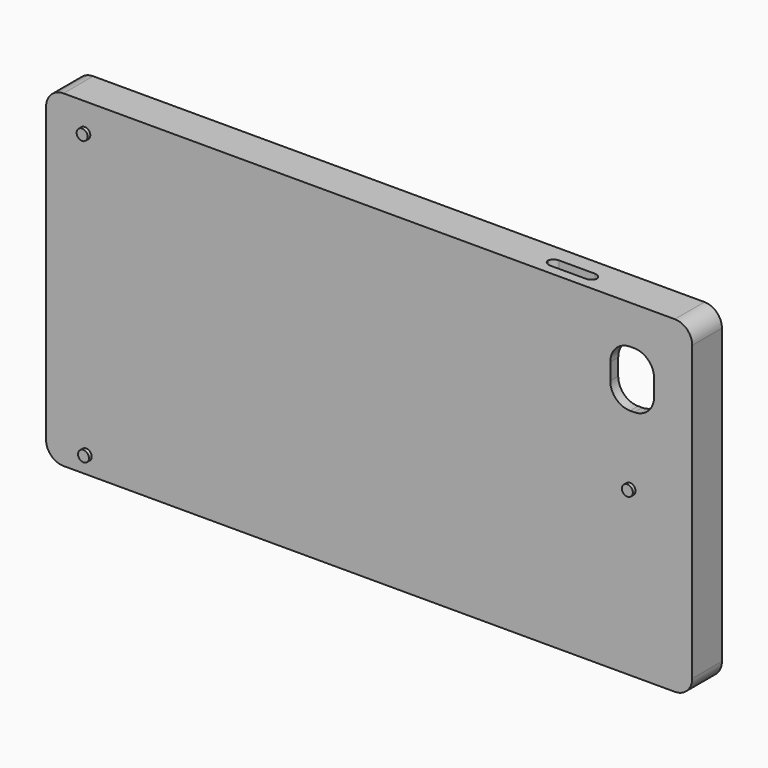
from build123d import *

# Parameters (mm, degrees)
F0_W         = 160.02
F0_H         = 78.74
F1_DEPTH     = 6.94228
F2_T         = 2.54
F3_T1_DEPTH  = 6.94228
F3_T3_DEPTH  = 31.70728
F4_W         = 11.2012028694
F4_H         = 14.4015364349
F6_DEPTH     = 25.4
F7_R         = 5.08
F8_W         = 2.54
F8_H         = 12.7
F8_H_2       = 17.78
F9_DEPTH     = 25.4
F10_W        = 10.3627294302
F10_H        = 4.2195547159
F10_W_2      = 10.414
F10_H_2      = 3.1508285339
F11_DEPTH    = 25.4
F12_T1_DEPTH = 2.54
F12_T3_DEPTH = 2.54
F13_W        = 12.7
F13_H        = 2.8448
F14_DEPTH    = 25.4
F15_T1_DEPTH = 2.54
F16_R        = 1.397
F17_DEPTH    = 0.86535


# Not quite as in the source:
# - a fillet or chamfer that OpenCascade refuses, or shapes differently, is made with other operations: its cross-section is extruded or revolved along the edge and cut away or added


with BuildPart() as f1:
    # F0 (on Front) → F1 (new body)
    with BuildSketch(Plane.XZ):
        with Locations((-0.5110458827, -0.4783872414)):
            Rectangle(F0_W, F0_H)
    extrude(amount=F1_DEPTH)

    # F2
    f2_openings = [f1.faces().sort_by_distance(p)[0] for p in [
        (-0.511046, 0, -0.478387),
    ]]
    offset(amount=F2_T, openings=f2_openings, kind=Kind.INTERSECTION)

    # F3: fillet of radius 4.445 on 8 edges, made by hand

    # F3_s2 → F3_t1 (join)
    with BuildSketch(Plane.XZ):
        with BuildLine():
            ThreePointArc((-76.0760458827, 38.8916127586), (-79.2191355251, 37.589702401), (-80.5210458827, 34.4466127586))
            Line((-80.5210458827, 34.4466127586), (-80.5210458827, 38.8916127586))
            Line((-80.5210458827, 38.8916127586), (-76.0760458827, 38.8916127586))
        make_face()
        with BuildLine():
            ThreePointArc((-80.5210458827, -35.4033872414), (-79.2191355251, -38.5464768837), (-76.0760458827, -39.8483872414))
            Line((-76.0760458827, -39.8483872414), (-80.5210458827, -39.8483872414))
            Line((-80.5210458827, -39.8483872414), (-80.5210458827, -35.4033872414))
        make_face()
        with BuildLine():
            ThreePointArc((79.4989541173, -35.4033872414), (78.1970437597, -38.5464768837), (75.0539541173, -39.8483872414))
            Line((75.0539541173, -39.8483872414), (79.4989541173, -39.8483872414))
            Line((79.4989541173, -39.8483872414), (79.4989541173, -35.4033872414))
        make_face()
        with BuildLine():
            ThreePointArc((79.4989541173, 34.4466127586), (78.1970437597, 37.589702401), (75.0539541173, 38.8916127586))
            Line((75.0539541173, 38.8916127586), (79.4989541173, 38.8916127586))
            Line((79.4989541173, 38.8916127586), (79.4989541173, 34.4466127586))
        make_face()
    extrude(amount=F3_T1_DEPTH)

    # F3_s4 → F3_t3 (cut)
    with BuildSketch(Plane.XZ.offset(-11.1125)):
        with BuildLine():
            ThreePointArc((77.5939541173, -42.3883872414), (80.7370437597, -41.0864768837), (82.0389541173, -37.9433872414))
            Line((82.0389541173, -37.9433872414), (82.0389541173, -42.3883872414))
            Line((82.0389541173, -42.3883872414), (77.5939541173, -42.3883872414))
        make_face()
        with BuildLine():
            ThreePointArc((82.0389541173, 36.9866127586), (80.7370437597, 40.129702401), (77.5939541173, 41.4316127586))
            Line((77.5939541173, 41.4316127586), (82.0389541173, 41.4316127586))
            Line((82.0389541173, 41.4316127586), (82.0389541173, 36.9866127586))
        make_face()
        with BuildLine():
            ThreePointArc((-83.0610458827, 36.9866127586), (-81.7591355251, 40.129702401), (-78.6160458827, 41.4316127586))
            Line((-78.6160458827, 41.4316127586), (-83.0610458827, 41.4316127586))
            Line((-83.0610458827, 41.4316127586), (-83.0610458827, 36.9866127586))
        make_face()
        with BuildLine():
            ThreePointArc((-83.0610458827, -37.9433872414), (-81.7591355251, -41.0864768837), (-78.6160458827, -42.3883872414))
            Line((-78.6160458827, -42.3883872414), (-83.0610458827, -42.3883872414))
            Line((-83.0610458827, -42.3883872414), (-83.0610458827, -37.9433872414))
        make_face()
    extrude(amount=F3_T3_DEPTH, mode=Mode.SUBTRACT)

    # F4 (on face) → F6 (cut)
    with BuildSketch(Plane(origin=(0, -6.94228, 0), x_dir=(-1, 0, 0), z_dir=(0, 1, 0))):
        with Locations((-66.6961297393, 24.3242625147)):
            Rectangle(F4_W, F4_H)
    extrude(amount=-F6_DEPTH, mode=Mode.SUBTRACT)

    # F7
    f7_edges = [f1.edges().sort_by_distance(p)[0] for p in [
        (72.296731, -8.21228, 31.525031),
        (72.296731, -8.21228, 17.123494),
        (61.095528, -8.21228, 31.525031),
        (61.095528, -8.21228, 17.123494),
    ]]
    fillet(f7_edges, radius=F7_R)

    # F8 (on face) → F9 (cut)
    with BuildSketch(Plane(origin=(-83.0610458827, 0, 0), x_dir=(0, -1, 0), z_dir=(-1, 0, 0))):
        with BuildLine():
            ThreePointArc((3.9402758845, -24.4620272314), (3.5303106613, -28.2545002504), (6.90014, -26.4669954777))
            ThreePointArc((6.90014, -26.4669954777), (6.5286447728, -25.256166139), (5.5420041155, -24.4620272314))
            ThreePointArc((5.5420041155, -24.4620272314), (4.74114, -24.7671066221), (3.9402758845, -24.4620272314))
        make_face()
        with BuildLine():
            ThreePointArc((3.9402758845, -24.4620272314), (4.74114, -24.3079954777), (5.5420041155, -24.4620272314))
            ThreePointArc((5.5420041155, -24.4620272314), (5.8395341143, -24.0557928593), (5.9448541617, -23.5633924603))
            ThreePointArc((5.9448541617, -23.5633924603), (4.2487396011, -22.4649983461), (3.9402758845, -24.4620272314))
        make_face()
        with Locations((4.74114, 0)):
            Rectangle(F8_W, F8_H)
        with Locations((4.74114, 20.6036127586)):
            Rectangle(F8_W, F8_H_2)
    extrude(amount=-F9_DEPTH, mode=Mode.SUBTRACT)

    # F10 (on face) → F11 (cut)
    with BuildSketch(Plane(origin=(0, 0, -42.3883872414), x_dir=(1, 0, 0), z_dir=(0, 0, -1))):
        with Locations((46.1594350636, 4.74114)):
            Rectangle(F10_W, F10_H)
        with Locations((27.6780048452, 4.74114)):
            Rectangle(F10_W_2, F10_H_2)
        with Locations((13.9850524713, 4.74114)):
            Rectangle(F10_W_2, F10_H_2)
    extrude(amount=-F11_DEPTH, mode=Mode.SUBTRACT)

    # F12: fillet of radius 1.5288490226 on 20 edges, made by hand

    # F12_s2 → F12_t1 (join)
    with BuildSketch(Plane.XY.offset(-42.3883872414)):
        with BuildLine():
            ThreePointArc((19.1920524713, -4.7877052443), (18.7442629599, -5.8687647556), (17.6632034486, -6.316554267))
            Line((17.6632034486, -6.316554267), (19.1920524713, -6.316554267))
            Line((19.1920524713, -6.316554267), (19.1920524713, -4.7877052443))
        make_face()
        with BuildLine():
            ThreePointArc((8.7780524713, -4.7877052443), (9.2258419826, -5.8687647556), (10.3069014939, -6.316554267))
            Line((10.3069014939, -6.316554267), (8.7780524713, -6.316554267))
            Line((8.7780524713, -6.316554267), (8.7780524713, -4.7877052443))
        make_face()
        with BuildLine():
            ThreePointArc((10.3069014939, -3.165725733), (9.2258419826, -3.6135152444), (8.7780524713, -4.6945747557))
            Line((8.7780524713, -4.6945747557), (8.7780524713, -3.165725733))
            Line((8.7780524713, -3.165725733), (10.3069014939, -3.165725733))
        make_face()
        with BuildLine():
            ThreePointArc((19.1920524713, -4.6945747557), (18.7442629599, -3.6135152444), (17.6632034486, -3.165725733))
            Line((17.6632034486, -3.165725733), (19.1920524713, -3.165725733))
            Line((19.1920524713, -3.165725733), (19.1920524713, -4.6945747557))
        make_face()
        with BuildLine():
            ThreePointArc((31.3561558226, -6.316554267), (32.4372153339, -5.8687647556), (32.8850048452, -4.7877052443))
            Line((32.8850048452, -4.7877052443), (32.8850048452, -6.316554267))
            Line((32.8850048452, -6.316554267), (31.3561558226, -6.316554267))
        make_face()
        with BuildLine():
            ThreePointArc((32.8850048452, -4.6945747557), (32.4372153339, -3.6135152444), (31.3561558226, -3.165725733))
            Line((31.3561558226, -3.165725733), (32.8850048452, -3.165725733))
            Line((32.8850048452, -3.165725733), (32.8850048452, -4.6945747557))
        make_face()
        with BuildLine():
            ThreePointArc((23.9998538678, -6.316554267), (22.9187943565, -5.8687647556), (22.4710048452, -4.7877052443))
            Line((22.4710048452, -4.7877052443), (22.4710048452, -6.316554267))
            Line((22.4710048452, -6.316554267), (23.9998538678, -6.316554267))
        make_face()
        with BuildLine():
            ThreePointArc((23.9998538678, -3.165725733), (22.9187943565, -3.6135152444), (22.4710048452, -4.6945747557))
            Line((22.4710048452, -4.6945747557), (22.4710048452, -3.165725733))
            Line((22.4710048452, -3.165725733), (23.9998538678, -3.165725733))
        make_face()
        with BuildLine():
            ThreePointArc((51.3407997787, -4.1602116647), (50.8930102674, -3.0791521534), (49.8119507561, -2.631362642))
            Line((49.8119507561, -2.631362642), (51.3407997787, -2.631362642))
            Line((51.3407997787, -2.631362642), (51.3407997787, -4.1602116647))
        make_face()
        with BuildLine():
            ThreePointArc((49.8119507561, -6.850917358), (50.8930102674, -6.4031278466), (51.3407997787, -5.3220683353))
            Line((51.3407997787, -5.3220683353), (51.3407997787, -6.850917358))
            Line((51.3407997787, -6.850917358), (49.8119507561, -6.850917358))
        make_face()
        with BuildLine():
            ThreePointArc((42.5069193711, -6.850917358), (41.4258598598, -6.4031278466), (40.9780703485, -5.3220683353))
            Line((40.9780703485, -5.3220683353), (40.9780703485, -6.850917358))
            Line((40.9780703485, -6.850917358), (42.5069193711, -6.850917358))
        make_face()
        with BuildLine():
            ThreePointArc((42.5069193711, -2.631362642), (41.4258598598, -3.0791521534), (40.9780703485, -4.1602116647))
            Line((40.9780703485, -4.1602116647), (40.9780703485, -2.631362642))
            Line((40.9780703485, -2.631362642), (42.5069193711, -2.631362642))
        make_face()
    extrude(amount=F12_T1_DEPTH)

    # F12_s4 → F12_t3 (join)
    with BuildSketch(Plane.YZ.offset(-83.0610458827)):
        with BuildLine():
            ThreePointArc((-4.9999890226, 11.7136127586), (-3.9189295113, 12.16140227), (-3.47114, 13.2424617813))
            Line((-3.47114, 13.2424617813), (-3.47114, 11.7136127586))
            Line((-3.47114, 11.7136127586), (-4.9999890226, 11.7136127586))
        make_face()
        with BuildLine():
            ThreePointArc((-6.01114, 27.964763736), (-5.5633504887, 29.0458232473), (-4.4822909774, 29.4936127586))
            Line((-4.4822909774, 29.4936127586), (-6.01114, 29.4936127586))
            Line((-6.01114, 29.4936127586), (-6.01114, 27.964763736))
        make_face()
        with BuildLine():
            ThreePointArc((-3.47114, 27.964763736), (-3.9189295113, 29.0458232473), (-4.9999890226, 29.4936127586))
            Line((-4.9999890226, 29.4936127586), (-3.47114, 29.4936127586))
            Line((-3.47114, 29.4936127586), (-3.47114, 27.964763736))
        make_face()
        with BuildLine():
            ThreePointArc((-6.01114, 13.2424617813), (-5.5633504887, 12.16140227), (-4.4822909774, 11.7136127586))
            Line((-4.4822909774, 11.7136127586), (-6.01114, 11.7136127586))
            Line((-6.01114, 11.7136127586), (-6.01114, 13.2424617813))
        make_face()
        with BuildLine():
            ThreePointArc((-6.01114, 4.8211509774), (-5.5633504887, 5.9022104887), (-4.4822909774, 6.35))
            Line((-4.4822909774, 6.35), (-6.01114, 6.35))
            Line((-6.01114, 6.35), (-6.01114, 4.8211509774))
        make_face()
        with BuildLine():
            ThreePointArc((-6.01114, -4.8211509774), (-5.5633504887, -5.9022104887), (-4.4822909774, -6.35))
            Line((-4.4822909774, -6.35), (-6.01114, -6.35))
            Line((-6.01114, -6.35), (-6.01114, -4.8211509774))
        make_face()
        with BuildLine():
            ThreePointArc((-4.9999890226, -6.35), (-3.9189295113, -5.9022104887), (-3.47114, -4.8211509774))
            Line((-3.47114, -4.8211509774), (-3.47114, -6.35))
            Line((-3.47114, -6.35), (-4.9999890226, -6.35))
        make_face()
        with BuildLine():
            ThreePointArc((-3.47114, 4.8211509774), (-3.9189295113, 5.9022104887), (-4.9999890226, 6.35))
            Line((-4.9999890226, 6.35), (-3.47114, 6.35))
            Line((-3.47114, 6.35), (-3.47114, 4.8211509774))
        make_face()
    extrude(amount=F12_T3_DEPTH)

    # F13 (on face) → F14 (cut)
    with BuildSketch(Plane.XY.offset(41.4316127586)):
        with Locations((48.2621807605, -5.5104298601)):
            Rectangle(F13_W, F13_H)
    extrude(amount=-F14_DEPTH, mode=Mode.SUBTRACT)

    # F15: fillet of radius 1.7551815441 on 4 edges, made by hand

    # F15_s2 → F15_t1 (join)
    with BuildSketch(Plane.XY.offset(38.8916127586)):
        with BuildLine():
            ThreePointArc((52.8569992164, -4.0880298601), (54.0980999884, -4.6021106321), (54.6121807605, -5.8432114042))
            Line((54.6121807605, -5.8432114042), (54.6121807605, -4.0880298601))
            Line((54.6121807605, -4.0880298601), (52.8569992164, -4.0880298601))
        make_face()
        with BuildLine():
            ThreePointArc((43.6673623046, -4.0880298601), (42.4262615326, -4.6021106321), (41.9121807605, -5.8432114042))
            Line((41.9121807605, -5.8432114042), (41.9121807605, -4.0880298601))
            Line((41.9121807605, -4.0880298601), (43.6673623046, -4.0880298601))
        make_face()
        with BuildLine():
            ThreePointArc((54.6121807605, -5.177648316), (54.0980999884, -6.418749088), (52.8569992164, -6.9328298601))
            Line((52.8569992164, -6.9328298601), (54.6121807605, -6.9328298601))
            Line((54.6121807605, -6.9328298601), (54.6121807605, -5.177648316))
        make_face()
        with BuildLine():
            ThreePointArc((43.6673623046, -6.9328298601), (42.4262615326, -6.418749088), (41.9121807605, -5.177648316))
            Line((41.9121807605, -5.177648316), (41.9121807605, -6.9328298601))
            Line((41.9121807605, -6.9328298601), (43.6673623046, -6.9328298601))
        make_face()
    extrude(amount=F15_T1_DEPTH)

    # F16 (on face) → F17 (join)
    with BuildSketch(Plane.XZ.offset(9.48228)):
        with Locations((66.1496967077, -0.4783872414)):
            Circle(F16_R)
        with Locations((-73.1634646654, 34.2442020774)):
            Circle(F16_R)
        with Locations((-72.7994458827, -37.9433872414)):
            Circle(F16_R)
    extrude(amount=F17_DEPTH)


solid = f1.part
